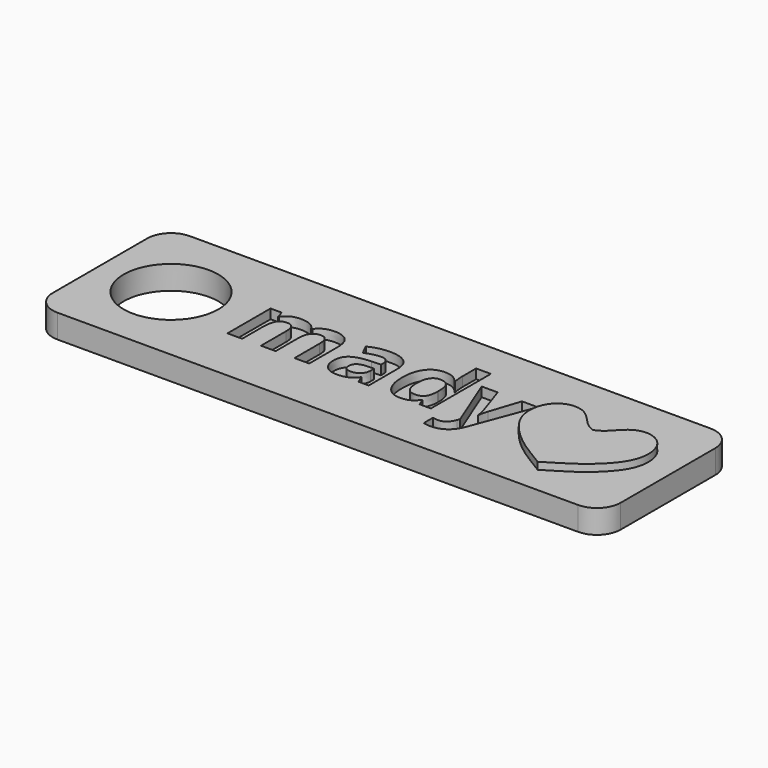
from build123d import *

# Parameters (mm, degrees)
F0_W         = 120
F0_H         = 35
F0_R         = 10
F1_DEPTH     = 5
F2_R         = 5
F3_TEXT_SIZE = 20.8333333333
F4_DEPTH     = 2
F6_DEPTH     = 1.5


# Not quite as in the source:
# - Text() gives the source's letters only with a copy of the font that has no kerning and outlines rounded to 1/6400 em; it was checked with that copy


with BuildPart() as f1:
    # F0 (on Top) → F1 (new body)
    with BuildSketch(Plane.XY):
        Rectangle(F0_W, F0_H)
        with Locations((-45, 0)):
            Circle(F0_R, mode=Mode.SUBTRACT)
    extrude(amount=F1_DEPTH)

    # F2
    f2_edges = [f1.edges().sort_by_distance(p)[0] for p in [
        (60, -17.5, 2.5),
        (60, 17.5, 2.5),
        (-60, -17.5, 2.5),
        (-60, 17.5, 2.5),
    ]]
    fillet(f2_edges, radius=F2_R)

    # F3 (on face) → F4 (cut)
    with BuildSketch(Plane.XY.offset(5)):
        with Locations((-30.1024175504, -5.7447621994)):
            Text('mady', F3_TEXT_SIZE, font='Open Sans', font_style=FontStyle.BOLD, text_align=(TextAlign.LEFT, TextAlign.BOTTOM))
    extrude(amount=-F4_DEPTH, mode=Mode.SUBTRACT)

    # F5 (on face) → F6 (join)
    with BuildSketch(Plane.XY.offset(5)):
        with BuildLine():
            add(Edge.make_bspline(
                [(41.9413633645, 2.728061052), (43.9636521041, 3.305856837), (46.035350201, 7.0890946873), (50.5747148192, 7.8626932604), (54.3609833724, 5.3248371498), (55.1706576898, -1.8916958999), (47.3749318138, -8.9064639421), (43.5065908895, -10.7773906443), (41.9413633645, -11.8612824008)],
                knots=[0, 0, 0, 0, 0.16750162, 0.3046914346, 0.440746448, 0.611895915, 0.828518195, 1, 1, 1, 1], degree=3))
            add(Edge.make_bspline(
                [(41.9413633645, 2.728061052), (39.9190746248, 3.305856837), (37.8473765279, 7.0890946873), (33.3080119097, 7.8626932604), (29.5217433565, 5.3248371498), (28.7120690391, -1.8916958999), (36.5077949151, -8.9064639421), (40.3761358394, -10.7773906443), (41.9413633645, -11.8612824008)],
                knots=[0, 0, 0, 0, 0.16750162, 0.3046914346, 0.440746448, 0.611895915, 0.828518195, 1, 1, 1, 1], degree=3))
        make_face()
    extrude(amount=F6_DEPTH)


solid = f1.part
